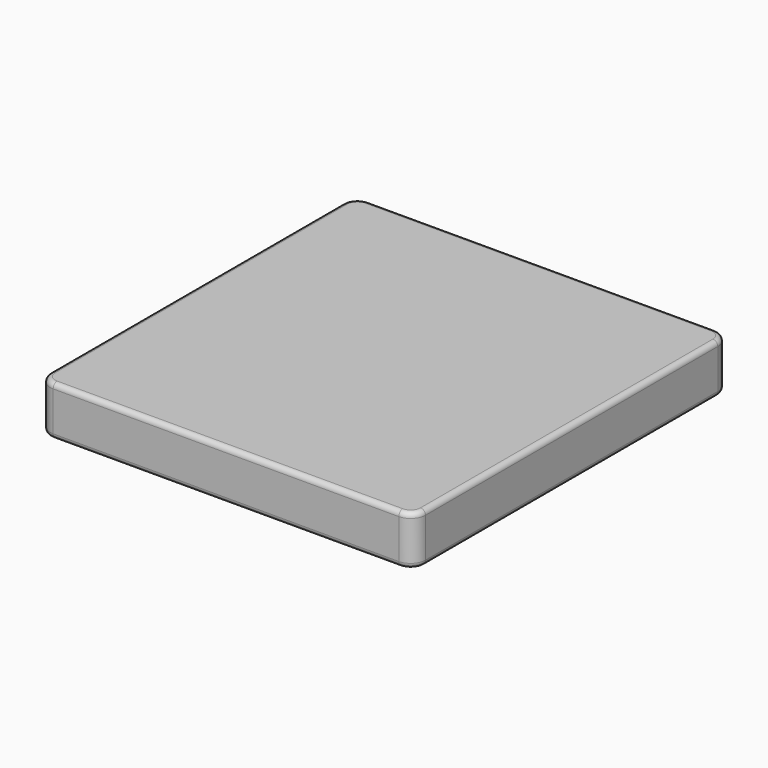
from build123d import *

# Parameters (mm, degrees)
F0_W         = 1930.4
F0_H         = 2032
F1_DEPTH     = 254
F2_R         = 25.4
F3_T1_DEPTH  = 254
F3_T4_ANGLE  = 90
F3_T6_ANGLE  = 90
F3_T8_ANGLE  = 90
F3_T10_ANGLE = 90
F3_T12_ANGLE = 90
F3_T14_ANGLE = 90
F3_T16_ANGLE = 90
F3_T18_ANGLE = 90


# Not quite as in the source:
# - a fillet or chamfer that OpenCascade refuses, or shapes differently, is made with other operations: its cross-section is extruded or revolved along the edge and cut away or added


with BuildPart() as f1:
    # F0 (on Top) → F1 (new body)
    with BuildSketch(Plane.XY):
        Rectangle(F0_W, F0_H)
    extrude(amount=F1_DEPTH)

    # F2
    f2_edges = [f1.edges().sort_by_distance(p)[0] for p in [
        (0, -1016, 254),
        (965.2, 0, 254),
        (0, 1016, 254),
        (-965.2, 0, 254),
        (0, -1016, 0),
        (965.2, 0, 0),
        (0, 1016, 0),
        (-965.2, 0, 0),
    ]]
    fillet(f2_edges, radius=F2_R)

    # F3: fillet of radius 76.2 on 4 edges, made by hand

    # F3_s2 → F3_t1 (cut)
    with BuildSketch(Plane.XY):
        with BuildLine():
            ThreePointArc((889, -1016), (942.8815367264, -993.6815367264), (965.2, -939.8))
            Line((965.2, -939.8), (965.2, -1016))
            Line((965.2, -1016), (889, -1016))
        make_face()
        with BuildLine():
            ThreePointArc((889, 1016), (942.8815367264, 993.6815367264), (965.2, 939.8))
            Line((965.2, 939.8), (965.2, 1016))
            Line((965.2, 1016), (889, 1016))
        make_face()
        with BuildLine():
            ThreePointArc((-965.2, -939.8), (-942.8815367264, -993.6815367264), (-889, -1016))
            Line((-889, -1016), (-965.2, -1016))
            Line((-965.2, -1016), (-965.2, -939.8))
        make_face()
        with BuildLine():
            ThreePointArc((-965.2, 939.8), (-942.8815367264, 993.6815367264), (-889, 1016))
            Line((-889, 1016), (-965.2, 1016))
            Line((-965.2, 1016), (-965.2, 939.8))
        make_face()
    extrude(amount=F3_T1_DEPTH, mode=Mode.SUBTRACT)

    # F3_s3 → F3_t4 (revolve, cut)
    with BuildSketch(Plane.XZ.offset(-939.8)):
        with BuildLine():
            ThreePointArc((-939.8, 0), (-957.7605122421, 7.4394877579), (-965.2, 25.4))
            Line((-965.2, 25.4), (-965.2, 0))
            Line((-965.2, 0), (-939.8, 0))
        make_face()
    revolve(axis=Axis((-889, 939.8, 0), (0, 0, -1)), revolution_arc=F3_T4_ANGLE, mode=Mode.SUBTRACT)

    # F3_s5 → F3_t6 (revolve, cut)
    with BuildSketch(Plane.YZ.offset(-889)):
        with BuildLine():
            ThreePointArc((990.6, 254), (1008.5605122421, 246.5605122421), (1016, 228.6))
            Line((1016, 228.6), (1016, 254))
            Line((1016, 254), (990.6, 254))
        make_face()
    revolve(axis=Axis((-889, 939.8, 254), (0, 0, 1)), revolution_arc=F3_T6_ANGLE, mode=Mode.SUBTRACT)

    # F3_s7 → F3_t8 (revolve, cut)
    with BuildSketch(Plane.YZ.offset(-889)):
        with BuildLine():
            ThreePointArc((-990.6, 0), (-1008.5605122421, 7.4394877579), (-1016, 25.4))
            Line((-1016, 25.4), (-1016, 0))
            Line((-1016, 0), (-990.6, 0))
        make_face()
    revolve(axis=Axis((-889, -939.8, 0), (0, 0, -1)), revolution_arc=F3_T8_ANGLE, mode=Mode.SUBTRACT)

    # F3_s9 → F3_t10 (revolve, cut)
    with BuildSketch(Plane.XZ.offset(939.8)):
        with BuildLine():
            ThreePointArc((-939.8, 254), (-957.7605122421, 246.5605122421), (-965.2, 228.6))
            Line((-965.2, 228.6), (-965.2, 254))
            Line((-965.2, 254), (-939.8, 254))
        make_face()
    revolve(axis=Axis((-889, -939.8, 254), (0, 0, 1)), revolution_arc=F3_T10_ANGLE, mode=Mode.SUBTRACT)

    # F3_s11 → F3_t12 (revolve, cut)
    with BuildSketch(Plane.YZ.offset(889)):
        with BuildLine():
            ThreePointArc((990.6, 0), (1008.5605122421, 7.4394877579), (1016, 25.4))
            Line((1016, 25.4), (1016, 0))
            Line((1016, 0), (990.6, 0))
        make_face()
    revolve(axis=Axis((889, 939.8, 0), (0, 0, -1)), revolution_arc=F3_T12_ANGLE, mode=Mode.SUBTRACT)

    # F3_s13 → F3_t14 (revolve, cut)
    with BuildSketch(Plane.XZ.offset(-939.8)):
        with BuildLine():
            ThreePointArc((939.8, 254), (957.7605122421, 246.5605122421), (965.2, 228.6))
            Line((965.2, 228.6), (965.2, 254))
            Line((965.2, 254), (939.8, 254))
        make_face()
    revolve(axis=Axis((889, 939.8, 254), (0, 0, 1)), revolution_arc=F3_T14_ANGLE, mode=Mode.SUBTRACT)

    # F3_s15 → F3_t16 (revolve, cut)
    with BuildSketch(Plane.XZ.offset(939.8)):
        with BuildLine():
            ThreePointArc((939.8, 0), (957.7605122421, 7.4394877579), (965.2, 25.4))
            Line((965.2, 25.4), (965.2, 0))
            Line((965.2, 0), (939.8, 0))
        make_face()
    revolve(axis=Axis((889, -939.8, 0), (0, 0, -1)), revolution_arc=F3_T16_ANGLE, mode=Mode.SUBTRACT)

    # F3_s17 → F3_t18 (revolve, cut)
    with BuildSketch(Plane.YZ.offset(889)):
        with BuildLine():
            ThreePointArc((-990.6, 254), (-1008.5605122421, 246.5605122421), (-1016, 228.6))
            Line((-1016, 228.6), (-1016, 254))
            Line((-1016, 254), (-990.6, 254))
        make_face()
    revolve(axis=Axis((889, -939.8, 254), (0, 0, 1)), revolution_arc=F3_T18_ANGLE, mode=Mode.SUBTRACT)


solid = f1.part
